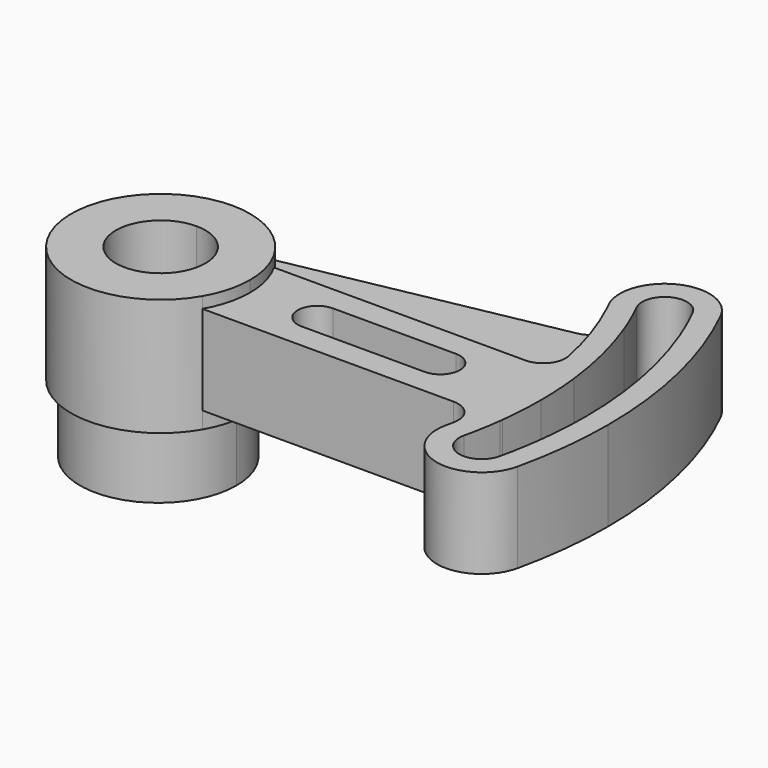
from build123d import *

# Parameters (mm, degrees)
F1_DEPTH     = 33.3248
F2_DEPTH     = 19.05
F3_DEPTH     = 30.1498
F5_DEPTH     = 4.7498
F6_DEPTH     = 22.225
F8_DEPTH     = 12.7
F9_T1_DEPTH  = 9.525
F9_T3_DEPTH  = 25.4
F9_T8_DEPTH  = 27.2571917505
F9_T13_DEPTH = 27.2317917505


# Not quite as in the source:
# - a fillet or chamfer that OpenCascade refuses, or shapes differently, is made with other operations: its cross-section is extruded or revolved along the edge and cut away or added


with BuildPart() as f1:
    # F0 (on Top) → F1 (new body)
    with BuildSketch(Plane.XY):
        with BuildLine():
            ThreePointArc((21.9970452561, 12.7), (12.7, 21.9970452561), (0, 25.4))
            ThreePointArc((0, 25.4), (-21.9970452561, -12.7), (21.9970452561, -12.7))
            ThreePointArc((21.9970452561, -12.7), (24.5345159877, -6.5740037456), (25.4, 0))
            ThreePointArc((25.4, 0), (24.5345159877, 6.5740037456), (21.9970452561, 12.7))
        make_face()
        with BuildLine():
            ThreePointArc((21.8425407432, -0.3824569867), (-16.232550455, -15.9620986388), (0, 21.8392519916))
            ThreePointArc((0, 21.8392519916), (15.4676319414, 15.1971846654), (21.8425407432, -0.3824569867))
        make_face(mode=Mode.SUBTRACT)
        with BuildLine():
            ThreePointArc((21.8425407432, -0.3824569867), (15.4676319414, 15.1971846654), (0, 21.8392519916))
            ThreePointArc((0, 21.8392519916), (-16.232550455, -15.9620986388), (21.8425407432, -0.3824569867))
        make_face()
        with BuildLine():
            ThreePointArc((0, 12.7), (8.9802561211, 8.9802561211), (12.7, 0))
            ThreePointArc((12.7, 0), (-8.9802561211, -8.9802561211), (0, 12.7))
        make_face(mode=Mode.SUBTRACT)
    extrude(amount=F1_DEPTH)

    # F0 (on Top) → F3 (join)
    with BuildSketch(Plane.XY):
        with BuildLine():
            Line((25.4, 12.7), (21.9970452561, 12.7))
            ThreePointArc((21.9970452561, 12.7), (24.5345159877, 6.5740037456), (25.4, 0))
            ThreePointArc((25.4, 0), (24.5345159877, -6.5740037456), (21.9970452561, -12.7))
            Line((21.9970452561, -12.7), (25.4, -12.7))
            Line((25.4, -12.7), (100.8031249516, -12.7))
            ThreePointArc((100.8031249516, -12.7), (101.4005855384, -6.3624879144), (101.6, 0))
            ThreePointArc((101.6, 0), (101.4005855384, 6.3624879144), (100.8031249516, 12.7))
            Line((100.8031249516, 12.7), (25.4, 12.7))
        make_face()
        with BuildLine():
            ThreePointArc((44.45, -5.5499), (38.9001, 0), (44.45, 5.5499))
            Line((44.45, 5.5499), (79.375, 5.5499))
            ThreePointArc((79.375, 5.5499), (83.2993719249, 3.9243719249), (84.9249, 0))
            ThreePointArc((84.9249, 0), (83.2993719249, -3.9243719249), (79.375, -5.5499))
            Line((79.375, -5.5499), (44.45, -5.5499))
        make_face(mode=Mode.SUBTRACT)
        with BuildLine():
            Line((107.2003381525, 12.7), (100.8031249516, 12.7))
            ThreePointArc((100.8031249516, 12.7), (101.4005855384, 6.3624879144), (101.6, 0))
            ThreePointArc((101.6, 0), (101.4005855384, -6.3624879144), (100.8031249516, -12.7))
            Line((100.8031249516, -12.7), (107.2003381525, -12.7))
            ThreePointArc((107.2003381525, -12.7), (107.762421566, -6.3610532321), (107.95, 0))
            ThreePointArc((107.95, 0), (107.762421566, 6.3610532321), (107.2003381525, 12.7))
        make_face()
        with BuildLine():
            ThreePointArc((91.0139318516, 45.1555556815), (91.4748276183, 44.2144310402), (91.9259920573, 43.2686027539))
            ThreePointArc((91.9259920573, 43.2686027539), (97.5691447351, 28.3341136382), (100.8031249516, 12.7))
            Line((100.8031249516, 12.7), (107.2003381525, 12.7))
            ThreePointArc((107.2003381525, 12.7), (104.8633855035, 25.6295314189), (100.9729543694, 38.1793790668))
            ThreePointArc((100.9729543694, 38.1793790668), (95.1042946416, 40.3981403326), (91.0139318516, 45.1555556815))
        make_face()
        with BuildLine():
            ThreePointArc((91.4835891574, 57.3058061184), (89.7001505826, 51.2905410623), (91.0139318516, 45.1555556815))
            ThreePointArc((91.0139318516, 45.1555556815), (95.1042946416, 40.3981403326), (100.9729543694, 38.1793790668))
            ThreePointArc((100.9729543694, 38.1793790668), (98.95897619, 43.1314679952), (96.7023027034, 47.9777776879))
            ThreePointArc((96.7023027034, 47.9777776879), (94.2084683161, 52.7064227352), (91.4835891574, 57.3058061184))
        make_face()
        with BuildLine():
            ThreePointArc((102.5883418008, 63.4984616078), (96.2051950503, 61.8918825067), (91.4835891574, 57.3058061184))
            ThreePointArc((91.4835891574, 57.3058061184), (94.2084683161, 52.7064227352), (96.7023027034, 47.9777776879))
            ThreePointArc((96.7023027034, 47.9777776879), (99.5684512872, 56.4883707973), (108.0790442979, 53.6222219202))
            ThreePointArc((108.0790442979, 53.6222219202), (105.4493808375, 58.6246584723), (102.5883418008, 63.4984616078))
        make_face()
        with BuildLine():
            ThreePointArc((113.7674145133, 56.4444452091), (109.1679535141, 61.5405062404), (102.5883418008, 63.4984616078))
            ThreePointArc((102.5883418008, 63.4984616078), (105.4493808375, 58.6246584723), (108.0790442979, 53.6222219202))
            ThreePointArc((108.0790442979, 53.6222219202), (110.4715620752, 48.5021285374), (112.6216847045, 43.2756124663))
            ThreePointArc((112.6216847044, 43.2756124663), (114.4576498997, 46.8404446919), (115.0906734034, 50.8))
            ThreePointArc((115.0906734034, 50.8), (114.7554340581, 53.6987400629), (113.7674145133, 56.4444452091))
        make_face()
        with BuildLine():
            ThreePointArc((115.0906734034, 50.8), (114.4576498997, 46.8404446919), (112.6216847044, 43.2756124663))
            ThreePointArc((112.6216847045, 43.2756124663), (118.6259431145, 22.0070016178), (120.65, 0))
            ThreePointArc((120.65, 0), (120.3936458808, -7.8608225729), (119.625672913, -15.6882401853))
            ThreePointArc((119.625672913, -15.6882401853), (122.957733543, -20.0447240945), (124.1420477199, -25.4))
            ThreePointArc((124.1420477199, -25.4), (124.0624104306, -26.8200158629), (123.8244973181, -28.2222228733))
            ThreePointArc((123.8244973181, -28.2222228733), (126.2036274427, -14.2001556434), (127, 0))
            ThreePointArc((127, 0), (123.6476074236, 28.9873968891), (113.7674145133, 56.4444452091))
            ThreePointArc((113.7674145133, 56.4444452091), (114.7554340581, 53.6987400629), (115.0906734034, 50.8))
        make_face()
        with BuildLine():
            ThreePointArc((124.1420477199, -25.4), (122.957733543, -20.0447240945), (119.625672913, -15.6882401853))
            ThreePointArc((119.625672913, -15.6882401853), (118.759763313, -21.2730138401), (117.6332727213, -26.8111105491))
            ThreePointArc((117.6332727213, -26.8111105491), (116.2486727134, -32.2903792542), (114.6090014612, -37.6987968517))
            ThreePointArc((114.6090014612, -37.6987968517), (120.546845886, -34.2539624098), (123.8244973181, -28.2222228733))
            ThreePointArc((123.8244973181, -28.2222228733), (124.0624104306, -26.8200158629), (124.1420477199, -25.4))
        make_face()
        with BuildLine():
            ThreePointArc((105.2508227996, -23.988889095), (103.9341328656, -29.1701649887), (102.3625461374, -34.2799015205))
            ThreePointArc((102.3625461374, -34.2799015205), (108.0271148048, -37.6322619815), (114.6090014612, -37.6987968517))
            ThreePointArc((114.6090014612, -37.6987968517), (116.2486727134, -32.2903792542), (117.6332727213, -26.8111105491))
            ThreePointArc((117.6332727213, -26.8111105491), (110.0309369928, -31.5912249609), (105.2508227996, -23.988889095))
        make_face()
        with BuildLine():
            ThreePointArc((107.1072287434, -13.462691072), (101.9216499986, -16.9945239737), (99.0595978685, -22.5777782371))
            ThreePointArc((99.0595978685, -22.5777782371), (99.2195781588, -28.8498170717), (102.3625461374, -34.2799015205))
            ThreePointArc((102.3625461374, -34.2799015205), (103.9341328656, -29.1701649887), (105.2508227996, -23.988889095))
            ThreePointArc((105.2508227996, -23.988889095), (106.309386815, -18.7487806272), (107.1072287434, -13.462691072))
        make_face()
        with BuildLine():
            Line((107.2003381525, -12.7), (100.8031249516, -12.7))
            ThreePointArc((100.8031249516, -12.7), (100.0533338724, -17.6604184834), (99.0595978685, -22.5777782371))
            ThreePointArc((99.0595978685, -22.5777782371), (101.9216499986, -16.9945239737), (107.1072287434, -13.462691072))
            ThreePointArc((107.1072287434, -13.462691072), (107.1544620239, -13.0814283766), (107.2003381525, -12.7))
        make_face()
    extrude(amount=F3_DEPTH)

    # F4 (on face) → F5 (cut)
    with BuildSketch(Plane(origin=(0, 0, 0), x_dir=(1, 0, 0), z_dir=(0, 0, -1))):
        with BuildLine():
            ThreePointArc((21.9970452561, 12.7), (24.5345159877, 6.5740037456), (25.4, 0))
            ThreePointArc((25.4, 0), (24.5345159877, -6.5740037456), (21.9970452561, -12.7))
            Line((21.9970452561, -12.7), (100.8031249516, -12.7))
            ThreePointArc((100.8031249516, -12.7), (97.2717152815, -29.3389401), (91.0139318516, -45.1555556815))
            ThreePointArc((91.0139318516, -45.1555556815), (96.7462286396, -62.1767413308), (113.7674145133, -56.4444452091))
            ThreePointArc((113.7674145133, -56.4444452091), (126.1134025906, -14.9803099778), (123.8244973181, 28.2222228733))
            ThreePointArc((123.8244973181, 28.2222228733), (108.6198254018, 37.7824497248), (99.0595978685, 22.5777782371))
            ThreePointArc((99.0595978685, 22.5777782371), (100.0533338724, 17.6604184834), (100.8031249516, 12.7))
            Line((100.8031249516, 12.7), (21.9970452561, 12.7))
        make_face()
        with BuildLine():
            Line((44.45, 5.5499), (79.375, 5.5499))
            ThreePointArc((79.375, 5.5499), (84.9249, 0), (79.375, -5.5499))
            Line((79.375, -5.5499), (44.45, -5.5499))
            ThreePointArc((44.45, -5.5499), (38.9001, 0), (44.45, 5.5499))
        make_face(mode=Mode.SUBTRACT)
        with BuildLine():
            ThreePointArc((117.6332727213, 26.8111105491), (119.8077324573, -14.23129451), (108.0790442979, -53.6222219202))
            ThreePointArc((108.0790442979, -53.6222219202), (99.5684512872, -56.4883707973), (96.7023027034, -47.9777776879))
            ThreePointArc((96.7023027034, -47.9777776879), (107.1963922297, -12.7332632479), (105.2508227996, 23.988889095))
            ThreePointArc((105.2508227996, 23.988889095), (110.0309369928, 31.5912249609), (117.6332727213, 26.8111105491))
        make_face(mode=Mode.SUBTRACT)
    extrude(amount=-F5_DEPTH, mode=Mode.SUBTRACT)

    # F0 (on Top) → F6 (join)
    with BuildSketch(Plane.XY):
        with BuildLine():
            Line((91.9259920573, 43.2686027539), (0, 25.4))
            ThreePointArc((0, 25.4), (12.7, 21.9970452561), (21.9970452561, 12.7))
            Line((21.9970452561, 12.7), (25.4, 12.7))
            Line((25.4, 12.7), (100.8031249516, 12.7))
            ThreePointArc((100.8031249516, 12.7), (97.5691447351, 28.3341136382), (91.9259920573, 43.2686027539))
        make_face()
    extrude(amount=F6_DEPTH)

    # F7 (on face) → F8 (cut)
    with BuildSketch(Plane(origin=(0, 0, 0), x_dir=(1, 0, 0), z_dir=(0, 0, -1))):
        with BuildLine():
            Line((100.8031249516, -12.7), (21.9970452561, -12.7))
            ThreePointArc((21.9970452561, -12.7), (12.7, -21.9970452561), (0, -25.4))
            Line((0, -25.4), (91.9259920573, -43.2686027539))
            ThreePointArc((91.9259920573, -43.2686027539), (97.5691447351, -28.3341136382), (100.8031249516, -12.7))
        make_face()
    extrude(amount=-F8_DEPTH, mode=Mode.SUBTRACT)

    # F9: fillet of radius 6.35 on 4 edges, made by hand

    # F9_s2 → F9_t1 (join)
    with BuildSketch(Plane.XY.offset(12.7)):
        with BuildLine():
            ThreePointArc((89.8183213038, 49.0039034869), (88.7059686824, 44.4242725365), (84.7437823747, 41.8725226155))
            Line((84.7437823747, 41.8725226155), (84.8649460867, 41.249189354))
            Line((84.8649460867, 41.249189354), (92.0471557694, 42.6452694924))
            Line((92.0471557694, 42.6452694924), (92.5005295077, 43.5390315211))
            ThreePointArc((92.5005295077, 43.5390315211), (91.5827689292, 45.4377778974), (90.4469389088, 49.0937083126))
            Line((90.4469389088, 49.0937083126), (89.8183213038, 49.0039034869))
        make_face()
    extrude(amount=F9_T1_DEPTH)

    # F9_s4 → F9_t3 (join)
    with BuildSketch(Plane.XY.offset(4.7498)):
        with BuildLine():
            ThreePointArc((99.5472631467, -20.32), (98.2442480497, -15.0339073716), (93.3255592, -12.7))
            Line((93.3255592, -12.7), (100.8031249516, -12.7))
            ThreePointArc((100.8031249516, -12.7), (100.247621432, -16.5219368483), (99.5472631467, -20.32))
        make_face()
    extrude(amount=F9_T3_DEPTH)


with BuildPart() as f2:
    # F0 (on Top) → F2 (new body)
    with BuildSketch(Plane.XY):
        with BuildLine():
            ThreePointArc((21.8425407432, -0.3824569867), (15.4676319414, 15.1971846654), (0, 21.8392519916))
            ThreePointArc((0, 21.8392519916), (-16.232550455, -15.9620986388), (21.8425407432, -0.3824569867))
        make_face()
        with BuildLine():
            ThreePointArc((0, 12.7), (8.9802561211, 8.9802561211), (12.7, 0))
            ThreePointArc((12.7, 0), (-8.9802561211, -8.9802561211), (0, 12.7))
        make_face(mode=Mode.SUBTRACT)
    extrude(amount=-F2_DEPTH)


with BuildPart() as f9_tool6:
    # F9_s7 → F9_t8 (new body)
    with BuildSketch(Plane.XY.offset(4.7498)):
        with BuildLine():
            ThreePointArc((99.5472631467, 20.32), (98.2442480497, 15.0339073716), (93.3255592, 12.7))
            Line((93.3255592, 12.7), (100.8031249516, 12.7))
            ThreePointArc((100.8031249516, 12.7), (100.247621432, 16.5219368483), (99.5472631467, 20.32))
        make_face()
    extrude(amount=F9_T8_DEPTH)

    split(bisect_by=Plane.XY.offset(30.1498), keep=Keep.BOTTOM)


with BuildPart() as f1_1:
    add(f1.part)

    # F9_t5: union F9_tool6
    add(f9_tool6.part)


with BuildPart() as f9_tool11:
    # F9_s12 → F9_t13 (new body)
    with BuildSketch(Plane.XY.offset(2.9180082495)):
        with BuildLine():
            ThreePointArc((99.5472631467, 20.32), (98.2442480497, 15.0339073716), (93.3255592, 12.7))
            Line((93.3255592, 12.7), (100.8031249516, 12.7))
            ThreePointArc((100.8031249516, 12.7), (100.247621432, 16.5219368483), (99.5472631467, 20.32))
        make_face()
    extrude(amount=F9_T13_DEPTH)

    split(bisect_by=Plane.XY.offset(4.7498), keep=Keep.TOP)


with BuildPart() as f1_2:
    add(f1_1.part)

    # F9_t10: union F9_tool11
    add(f9_tool11.part)


solid = Compound([f2.part, f1_2.part])
